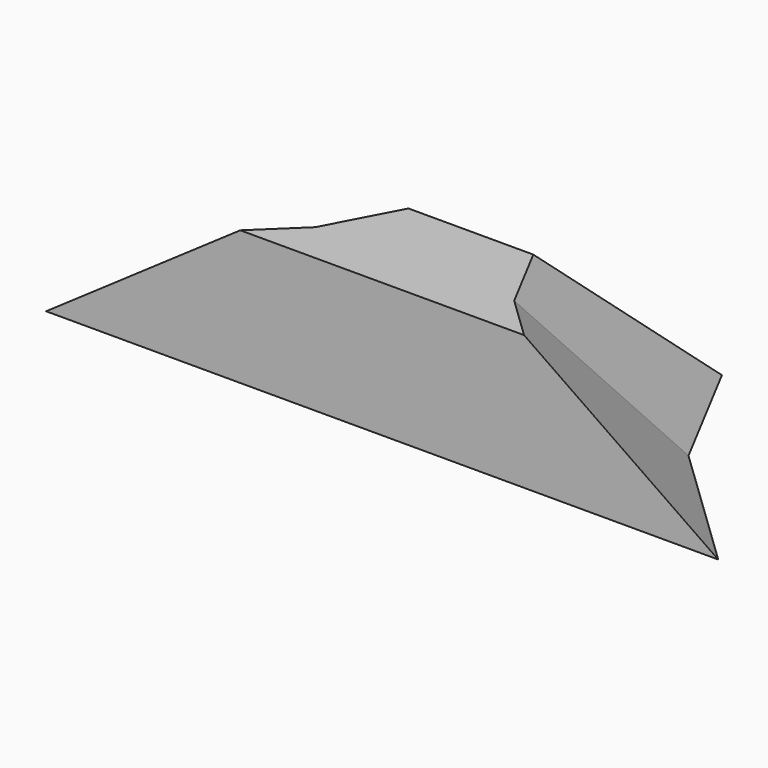
from build123d import *

# Parameters (mm, degrees)
F1_DEPTH = 20
F2_SIZE  = 19.99999


# Not quite as in the source:
# - a fillet or chamfer is up to 0.001 mm smaller than in the source, because OpenCascade refuses the exact size


with BuildPart() as f1:
    # F0 (on Top) → F1 (new body)
    with BuildSketch(Plane.XY):
        Polygon((-30.9781403543, -6.75), (-50, -25), (50, -25), (30.9781403543, -6.75), (21.3486810742, 11.5), (-21.3486810742, 11.5), align=None)
    extrude(amount=F1_DEPTH)

    # F2 (size 20 in the source; OpenCascade refuses exactly that, so slightly less here)
    f2_edges = [f1.edges().sort_by_distance(p)[0] for p in [
        (0, 11.5, 20),
        (26.163411, 2.375, 20),
        (40.48907, -15.875, 20),
        (-40.48907, -15.875, 20),
        (-26.163411, 2.375, 20),
    ]]
    chamfer(f2_edges, length=F2_SIZE)


solid = f1.part
